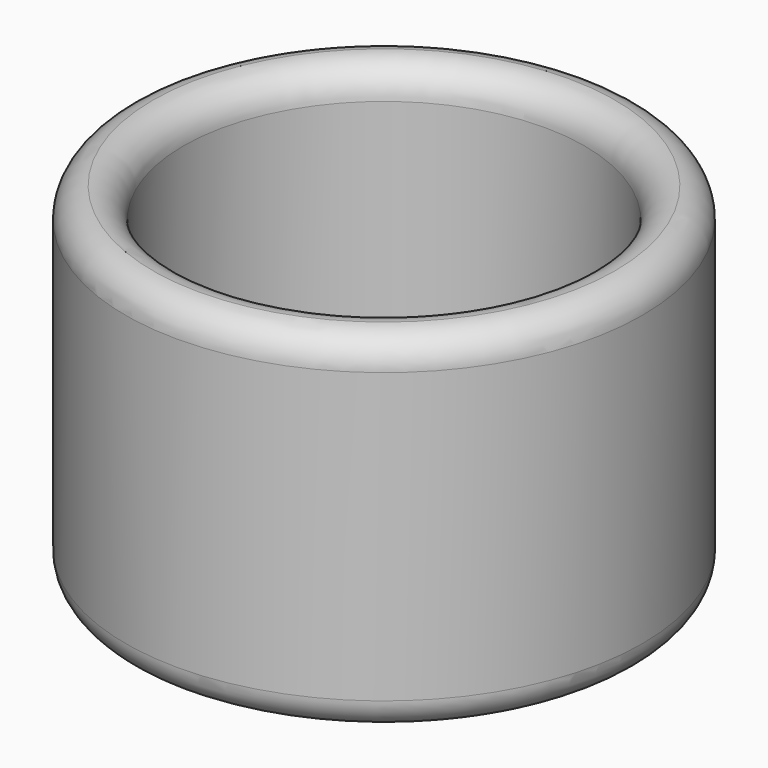
from build123d import *

# Parameters (mm, degrees)
F0_R     = 8.5
F1_DEPTH = 3.5
F2_R     = 8.5
F2_R_2   = 6.6
F3_DEPTH = 8
F4_R     = 1


# Not quite as in the source:
# - a fillet or chamfer that OpenCascade refuses, or shapes differently, is made with other operations: its cross-section is extruded or revolved along the edge and cut away or added
# - a feature names something its author has since deleted; it is built from what else it names


with BuildPart() as f1:
    # F0 (on Top) → F1 (new body)
    with BuildSketch(Plane.XY):
        Circle(F0_R)
    extrude(amount=-F1_DEPTH)

    # F2 (on face) → F3 (join)
    with BuildSketch(Plane.XY):
        Circle(F2_R)
        Circle(F2_R_2, mode=Mode.SUBTRACT)
    extrude(amount=F3_DEPTH)

    # F4
    f4_edges = [f1.edges().sort_by_distance(p)[0] for p in [
        (-6.6, 0, 8),
        (-8.5, 0, -3.5),
    ]]
    fillet(f4_edges, radius=F4_R)

    # F5: fillet of radius 1 on 1 edges, made by hand

    # F5_s1 → F5_t2 (revolve, cut)
    with BuildSketch(Plane.XZ):
        with BuildLine():
            ThreePointArc((8.5, 7.0050125629), (8.2416198487, 7.6758329561), (7.6, 8))
            Line((7.6, 8), (8.5, 8))
            Line((8.5, 8), (8.5, 7.0050125629))
        make_face()
    revolve(axis=Axis((0, 0, 8), (0, 0, 1)), mode=Mode.SUBTRACT)


solid = f1.part
